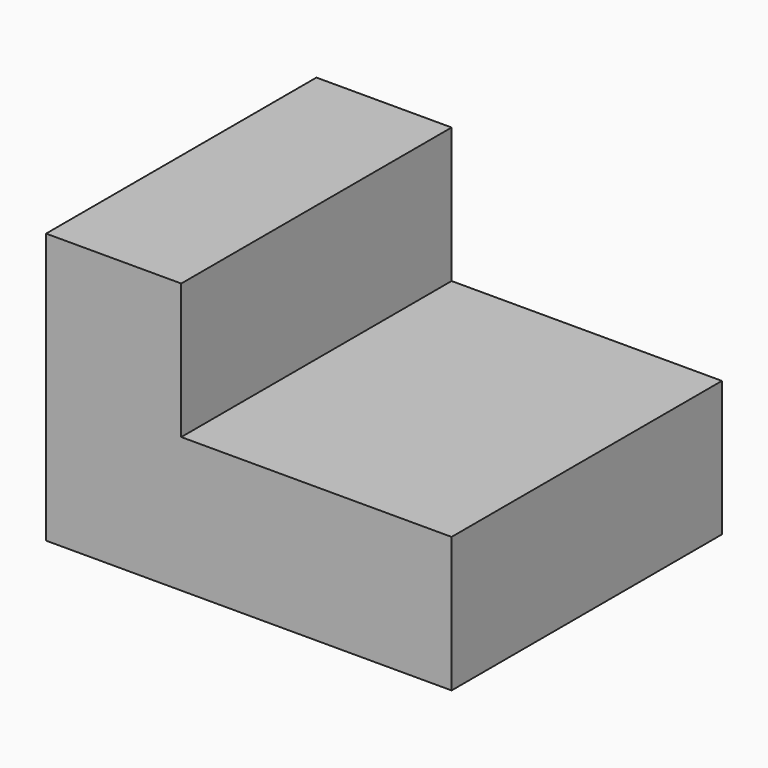
from build123d import *

# Parameters (mm, degrees)
F1_DEPTH = 127


# Not quite as in the source:
# - a feature names something its author has since deleted; it is built from what else it names


with BuildPart() as f1:
    # F0 (on Front) → F1 (new body)
    with BuildSketch(Plane.XZ):
        Polygon((-75.8873522282, 45.2570778489), (-75.8873522282, -56.3429221511), (76.5126477718, -56.3429221511), (76.5126477718, -5.5429221511), (-25.0873522282, -5.5429221511), (-25.0873522282, 45.2570778489), align=None)
    extrude(amount=F1_DEPTH)


solid = f1.part
